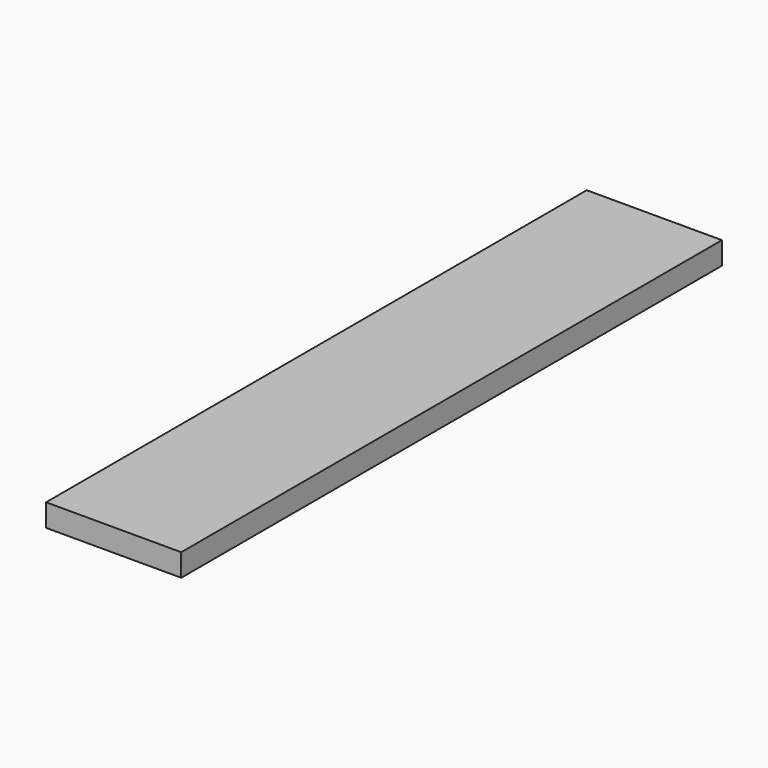
from build123d import *

# Parameters (mm, degrees)
F1_DEPTH = 150


# Not quite as in the source:
# - a feature names something its author has since deleted; it is built from what else it names


with BuildPart() as f1:
    # F0 (on Front) → F1 (new body)
    with BuildSketch(Plane.XZ):
        Polygon((30, -15), (3, -15), (0, -15), (0, -20), (30, -20), align=None)
    extrude(amount=F1_DEPTH)


solid = f1.part
